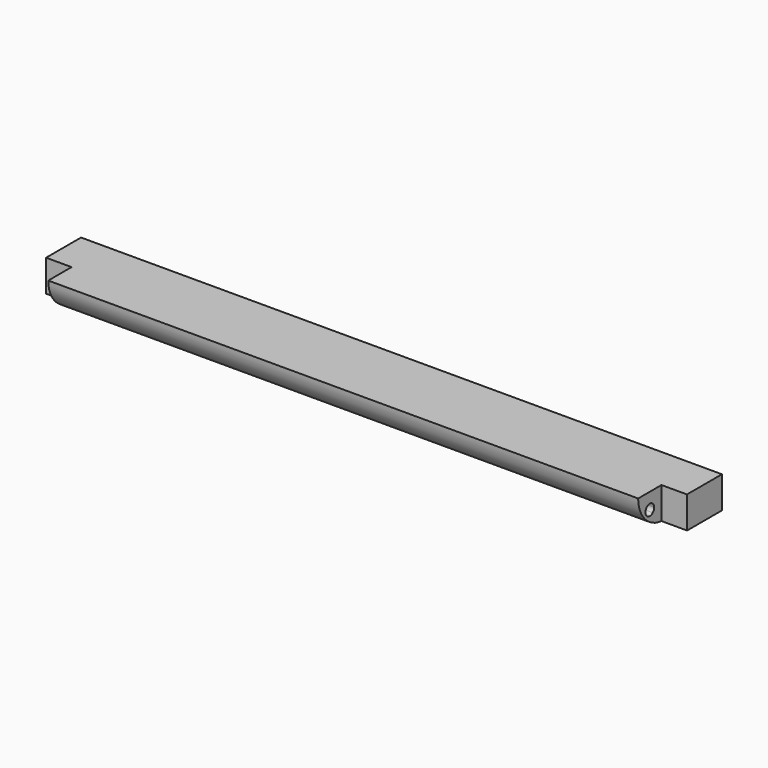
from build123d import *

# Parameters (mm, degrees)
F0_W     = 127
F0_H     = 55.5625
F1_DEPTH = 1117.6
F2_W     = 44.45
F2_H     = 50.8
F3_DEPTH = 55.5635
F5_DEPTH = 1073.151
F6_R     = 55.56249


# Not quite as in the source:
# - a fillet or chamfer is up to 0.001 mm smaller than in the source, because OpenCascade refuses the exact size


with BuildPart() as f1:
    # F0 (on Right) → F1 (new body)
    with BuildSketch(Plane.YZ):
        Rectangle(F0_W, F0_H)
    extrude(amount=F1_DEPTH)

    # F2 (on face) → F3 (cut, through all)
    with BuildSketch(Plane.XY.offset(27.78125)):
        with Locations((22.225, -38.1)):
            Rectangle(F2_W, F2_H)
        with Locations((1095.375, -38.1)):
            Rectangle(F2_W, F2_H)
    extrude(amount=-F3_DEPTH, mode=Mode.SUBTRACT)

    # F4 (on face) → F5 (cut, through all)
    with BuildSketch(Plane.YZ.offset(1073.15)):
        with BuildLine():
            Line((-38.1, 0), (-44.5271766257, -7.0297244343))
            ThreePointArc((-44.5271766257, -7.0297244343), (-38.1, -9.525), (-31.6728233743, -7.0297244343))
            Line((-31.6728233743, -7.0297244343), (-38.1, 0))
        make_face()
        with BuildLine():
            ThreePointArc((-44.5271766257, 7.0297244343), (-47.625, 0), (-44.5271766257, -7.0297244343))
            Line((-44.5271766257, -7.0297244343), (-38.1, 0))
            Line((-38.1, 0), (-44.5271766257, 7.0297244343))
        make_face()
        with BuildLine():
            Line((-44.5271766257, 7.0297244343), (-38.1, 0))
            Line((-38.1, 0), (-31.6728233743, 7.0297244343))
            ThreePointArc((-31.6728233743, 7.0297244343), (-38.1, 9.525), (-44.5271766257, 7.0297244343))
        make_face()
        with BuildLine():
            Line((-31.6728233743, 7.0297244343), (-38.1, 0))
            Line((-38.1, 0), (-31.6728233743, -7.0297244343))
            ThreePointArc((-31.6728233743, -7.0297244343), (-29.3837943359, -3.8410133845), (-28.575, 0))
            ThreePointArc((-28.575, 0), (-29.3837943359, 3.8410133845), (-31.6728233743, 7.0297244343))
        make_face()
    extrude(amount=-F5_DEPTH, mode=Mode.SUBTRACT)

    # F6 (radius 55.5625 in the source; OpenCascade refuses exactly that, so slightly less here)
    f6_edges = [f1.edges().sort_by_distance(p)[0] for p in [
        (558.8, -63.5, -27.78125),
    ]]
    fillet(f6_edges, radius=F6_R)


solid = f1.part
